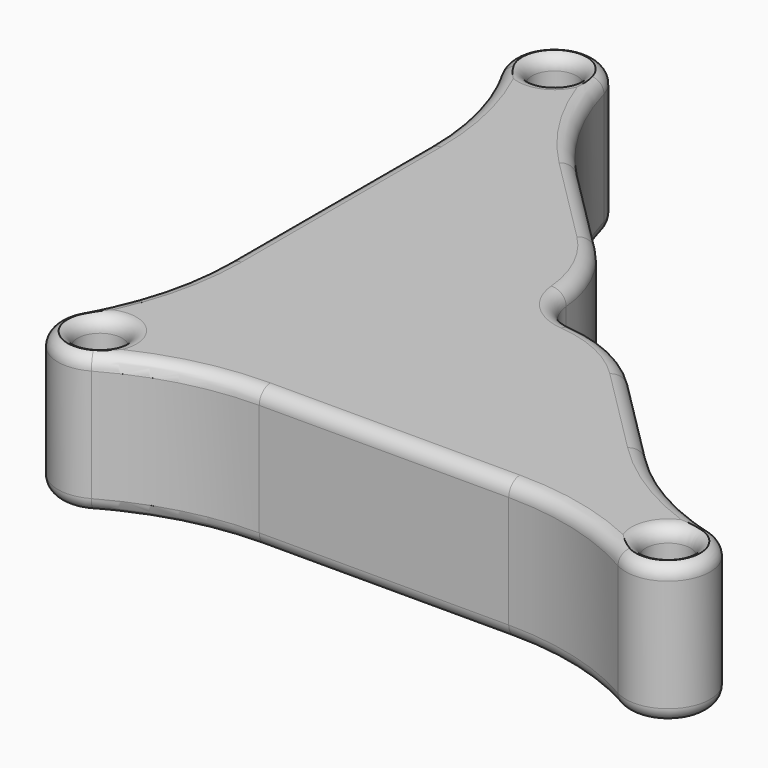
from build123d import *

# Parameters (mm, degrees)
F0_R          = 1.6
F1_DEPTH      = 10
F2_T3_ANGLE   = 29.591845794
F2_T6_ANGLE   = 194.1836915879
F2_T9_ANGLE   = 29.591845794
F2_T12_DEPTH  = 17.7843666168
F2_T15_ANGLE  = 29.591845794
F2_T18_ANGLE  = 149.1836915879
F2_T21_ANGLE  = 29.591845794
F2_T24_DEPTH  = 17.7843666168
F2_T27_ANGLE  = 29.591845794
F2_T30_ANGLE  = 194.1836915879
F2_T33_ANGLE  = 29.591845794
F2_T36_DEPTH  = 8.9733840835
F2_T39_ANGLE  = 39.7151372318
F2_T42_ANGLE  = 79.4302744637
F2_T45_ANGLE  = 39.7151372318
F2_T48_DEPTH  = 8.9733840835
F2_T60_ANGLE  = 29.591845794
F2_T63_ANGLE  = 194.1836915879
F2_T66_ANGLE  = 29.591845794
F2_T69_DEPTH  = 17.7843666168
F2_T72_ANGLE  = 29.591845794
F2_T75_ANGLE  = 149.1836915879
F2_T78_ANGLE  = 29.591845794
F2_T81_DEPTH  = 17.7843666168
F2_T84_ANGLE  = 29.591845794
F2_T87_ANGLE  = 194.1836915879
F2_T90_ANGLE  = 29.591845794
F2_T93_DEPTH  = 8.9733840835
F2_T96_ANGLE  = 39.7151372318
F2_T99_ANGLE  = 79.4302744637
F2_T102_ANGLE = 39.7151372318
F2_T105_DEPTH = 8.9733840835


# Not quite as in the source:
# - a fillet or chamfer that OpenCascade refuses, or shapes differently, is made with other operations: its cross-section is extruded or revolved along the edge and cut away or added


with BuildPart() as f1:
    # F0 (on Top) → F1 (new body)
    with BuildSketch(Plane.XY):
        with BuildLine():
            Line((11.3578166916, 0), (29.1421833084, 0))
            ThreePointArc((29.1421833084, 0), (34.249722493, -0.6631687322), (39.0185456489, -2.6086956522))
            ThreePointArc((39.0185456489, -2.6086956522), (43.2716385975, -1.1480502971), (41.297079968, 2.8921728034))
            ThreePointArc((41.297079968, 2.8921728034), (36.5493174981, 4.8885447172), (32.4688107979, 8.0311892021))
            Line((32.4688107979, 8.0311892021), (26.1236700622, 14.3763299378))
            ThreePointArc((26.1236700622, 14.3763299378), (23.3013016609, 16.3578061506), (19.9736774424, 17.2627527983))
            ThreePointArc((19.9736774424, 17.2627527983), (18.1286796564, 18.1286796564), (17.2627527983, 19.9736774424))
            ThreePointArc((17.2627527983, 19.9736774424), (16.3578061506, 23.3013016609), (14.3763299378, 26.1236700622))
            Line((14.3763299378, 26.1236700622), (8.0311892021, 32.4688107979))
            ThreePointArc((8.0311892021, 32.4688107979), (4.8885447172, 36.5493174981), (2.8921728034, 41.297079968))
            ThreePointArc((2.8921728034, 41.297079968), (-1.1480502971, 43.2716385975), (-2.6086956522, 39.0185456489))
            ThreePointArc((-2.6086956522, 39.0185456489), (-0.6631687322, 34.249722493), (0, 29.1421833084))
            Line((0, 29.1421833084), (0, 11.3578166916))
            ThreePointArc((0, 11.3578166916), (-0.6631687322, 6.250277507), (-2.6086956522, 1.4814543511))
            ThreePointArc((-2.6086956522, 1.4814543511), (-2.1213203436, -2.1213203436), (1.4814543511, -2.6086956522))
            ThreePointArc((1.4814543511, -2.6086956522), (6.250277507, -0.6631687322), (11.3578166916, 0))
        make_face()
        Circle(F0_R, mode=Mode.SUBTRACT)
        with Locations((40.5, 0)):
            Circle(F0_R, mode=Mode.SUBTRACT)
        with Locations((0, 40.5)):
            Circle(F0_R, mode=Mode.SUBTRACT)
    extrude(amount=F1_DEPTH)

    # F2: fillet of radius 1 on 38 edges, made by hand


with BuildPart() as f2_tool1:
    # F2_s2 → F2_t3 (revolve)
    with BuildSketch(Plane(origin=(-12.2188107979, 12.2188107979, 0), x_dir=(0, 0, 1), z_dir=(0.7071067812, -0.7071067812, 0))):
        with BuildLine():
            ThreePointArc((9, -28.6378246381), (9.7071067812, -28.3449314192), (10, -27.6378246381))
            Line((10, -27.6378246381), (10, -28.6378246381))
            Line((10, -28.6378246381), (9, -28.6378246381))
        make_face()
    revolve(axis=Axis((22.1733248258, 46.6109464216, 10), (0, 0, -1)), revolution_arc=F2_T3_ANGLE)


with BuildPart() as f2_tool4:
    # F2_s5 → F2_t6 (revolve)
    with BuildSketch(Plane(origin=(-10.3738185255, 37.6409858605, 0), x_dir=(0, 0, 1), z_dir=(0.2656933227, -0.9640576011, 0))):
        with BuildLine():
            ThreePointArc((9, -13.7605795685), (9.7071067812, -13.4676863497), (10, -12.7605795685))
            Line((10, -12.7605795685), (10, -13.7605795685))
            Line((10, -13.7605795685), (9, -13.7605795685))
        make_face()
    revolve(axis=Axis((0, 40.5, 10), (0, 0, 1)), revolution_arc=F2_T6_ANGLE)


with BuildPart() as f2_tool7:
    # F2_s8 → F2_t9 (revolve)
    with BuildSketch(Plane(origin=(-17.3909858605, 30.6238185255, 0), x_dir=(0, 0, 1), z_dir=(-0.493818117, 0.8695652174, 0))):
        with BuildLine():
            ThreePointArc((9, 16.9996337396), (9.7071067812, 17.2925269584), (10, 17.9996337396))
            Line((10, 17.9996337396), (10, 16.9996337396))
            Line((10, 16.9996337396), (9, 16.9996337396))
        make_face()
    revolve(axis=Axis((-20, 29.1421833084, 10), (0, 0, -1)), revolution_arc=F2_T9_ANGLE)


with BuildPart() as f2_tool10:
    # F2_s11 → F2_t12 (new body)
    with BuildSketch(Plane.XZ.offset(-29.1421833084)):
        with BuildLine():
            ThreePointArc((0, 9), (0.2928932188, 9.7071067812), (1, 10))
            Line((1, 10), (0, 10))
            Line((0, 10), (0, 9))
        make_face()
    extrude(amount=F2_T12_DEPTH)


with BuildPart() as f2_tool13:
    # F2_s14 → F2_t15 (revolve)
    with BuildSketch(Plane.XZ.offset(-11.3578166916)):
        with BuildLine():
            ThreePointArc((0, 9), (0.2928932188, 9.7071067812), (1, 10))
            Line((1, 10), (0, 10))
            Line((0, 10), (0, 9))
        make_face()
    revolve(axis=Axis((-20, 11.3578166916, 10), (0, 0, -1)), revolution_arc=F2_T15_ANGLE)


with BuildPart() as f2_tool16:
    # F2_s17 → F2_t18 (revolve)
    with BuildSketch(Plane(origin=(0, 0, 0), x_dir=(0, 0, 1), z_dir=(0.493818117, 0.8695652174, 0))):
        with BuildLine():
            ThreePointArc((9, -3), (9.7071067812, -2.7071067812), (10, -2))
            Line((10, -2), (10, -3))
            Line((10, -3), (9, -3))
        make_face()
    revolve(axis=Axis((0, 0, 10), (0, 0, 1)), revolution_arc=F2_T18_ANGLE)


with BuildPart() as f2_tool19:
    # F2_s20 → F2_t21 (revolve)
    with BuildSketch(Plane(origin=(0, 0, 0), x_dir=(0, 0, 1), z_dir=(-0.8695652174, -0.493818117, 0))):
        with BuildLine():
            ThreePointArc((9, -3), (9.7071067812, -2.7071067812), (10, -2))
            Line((10, -2), (10, -3))
            Line((10, -3), (9, -3))
        make_face()
    revolve(axis=Axis((11.3578166916, -20, 10), (0, 0, -1)), revolution_arc=F2_T21_ANGLE)


with BuildPart() as f2_tool22:
    # F2_s23 → F2_t24 (new body)
    with BuildSketch(Plane.YZ.offset(11.3578166916)):
        with BuildLine():
            ThreePointArc((0, 9), (0.2928932188, 9.7071067812), (1, 10))
            Line((1, 10), (0, 10))
            Line((0, 10), (0, 9))
        make_face()
    extrude(amount=F2_T24_DEPTH)


with BuildPart() as f2_tool25:
    # F2_s26 → F2_t27 (revolve)
    with BuildSketch(Plane.YZ.offset(29.1421833084)):
        with BuildLine():
            ThreePointArc((0, 9), (0.2928932188, 9.7071067812), (1, 10))
            Line((1, 10), (0, 10))
            Line((0, 10), (0, 9))
        make_face()
    revolve(axis=Axis((29.1421833084, -20, 10), (0, 0, -1)), revolution_arc=F2_T27_ANGLE)


with BuildPart() as f2_tool28:
    # F2_s29 → F2_t30 (revolve)
    with BuildSketch(Plane(origin=(30.6238185255, -17.3909858605, 0), x_dir=(0, 0, 1), z_dir=(-0.8695652174, 0.493818117, 0))):
        with BuildLine():
            ThreePointArc((9, 16.9996337396), (9.7071067812, 17.2925269584), (10, 17.9996337396))
            Line((10, 17.9996337396), (10, 16.9996337396))
            Line((10, 16.9996337396), (9, 16.9996337396))
        make_face()
    revolve(axis=Axis((40.5, 0, 10), (0, 0, 1)), revolution_arc=F2_T30_ANGLE)


with BuildPart() as f2_tool31:
    # F2_s32 → F2_t33 (revolve)
    with BuildSketch(Plane(origin=(37.6409858605, -10.3738185255, 0), x_dir=(0, 0, 1), z_dir=(0.9640576011, -0.2656933227, 0))):
        with BuildLine():
            ThreePointArc((9, -13.7605795685), (9.7071067812, -13.4676863497), (10, -12.7605795685))
            Line((10, -12.7605795685), (10, -13.7605795685))
            Line((10, -13.7605795685), (9, -13.7605795685))
        make_face()
    revolve(axis=Axis((46.6109464216, 22.1733248258, 10), (0, 0, -1)), revolution_arc=F2_T33_ANGLE)


with BuildPart() as f2_tool34:
    # F2_s35 → F2_t36 (new body)
    with BuildSketch(Plane(origin=(12.2188107979, -12.2188107979, 0), x_dir=(0, 0, 1), z_dir=(-0.7071067812, 0.7071067812, 0))):
        with BuildLine():
            ThreePointArc((9, 28.6378246381), (9.7071067812, 28.3449314192), (10, 27.6378246381))
            Line((10, 27.6378246381), (10, 28.6378246381))
            Line((10, 28.6378246381), (9, 28.6378246381))
        make_face()
    extrude(amount=F2_T36_DEPTH)


with BuildPart() as f2_tool37:
    # F2_s38 → F2_t39 (revolve)
    with BuildSketch(Plane(origin=(5.8736700622, -5.8736700622, 0), x_dir=(0, 0, 1), z_dir=(0.7071067812, -0.7071067812, 0))):
        with BuildLine():
            ThreePointArc((9, -28.6378246381), (9.7071067812, -28.3449314192), (10, -27.6378246381))
            Line((10, -27.6378246381), (10, -28.6378246381))
            Line((10, -28.6378246381), (9, -28.6378246381))
        make_face()
    revolve(axis=Axis((19.0526022504, 7.3052621259, 10), (0, 0, 1)), revolution_arc=F2_T39_ANGLE)


with BuildPart() as f2_tool40:
    # F2_s41 → F2_t42 (revolve)
    with BuildSketch(Plane(origin=(18.2209546286, -1.6854516701, 0), x_dir=(0, 0, 1), z_dir=(0.9957490672, -0.0921075192, 0))):
        with BuildLine():
            ThreePointArc((9, -19.0290958754), (9.7071067812, -18.7362026566), (10, -18.0290958754))
            Line((10, -18.0290958754), (10, -19.0290958754))
            Line((10, -19.0290958754), (9, -19.0290958754))
        make_face()
    revolve(axis=Axis((20.25, 20.25, 10), (0, 0, -1)), revolution_arc=F2_T42_ANGLE)


with BuildPart() as f2_tool43:
    # F2_s44 → F2_t45 (revolve)
    with BuildSketch(Plane(origin=(-1.6854516701, 18.2209546286, 0), x_dir=(0, 0, 1), z_dir=(0.0921075192, -0.9957490672, 0))):
        with BuildLine():
            ThreePointArc((9, -19.0290958754), (9.7071067812, -18.7362026566), (10, -18.0290958754))
            Line((10, -18.0290958754), (10, -19.0290958754))
            Line((10, -19.0290958754), (9, -19.0290958754))
        make_face()
    revolve(axis=Axis((7.3052621259, 19.0526022504, 10), (0, 0, 1)), revolution_arc=F2_T45_ANGLE)


with BuildPart() as f2_tool46:
    # F2_s47 → F2_t48 (new body)
    with BuildSketch(Plane(origin=(-5.8736700622, 5.8736700622, 0), x_dir=(0, 0, 1), z_dir=(-0.7071067812, 0.7071067812, 0))):
        with BuildLine():
            ThreePointArc((9, 28.6378246381), (9.7071067812, 28.3449314192), (10, 27.6378246381))
            Line((10, 27.6378246381), (10, 28.6378246381))
            Line((10, 28.6378246381), (9, 28.6378246381))
        make_face()
    extrude(amount=F2_T48_DEPTH)


with BuildPart() as f2_tool49:
    # F2_s50 → F2_t51 (revolve)
    with BuildSketch(Plane.XZ):
        with BuildLine():
            ThreePointArc((1.6, 9), (1.8928932188, 9.7071067812), (2.6, 10))
            Line((2.6, 10), (1.6, 10))
            Line((1.6, 10), (1.6, 9))
        make_face()
    revolve(axis=Axis((0, 0, 10), (0, 0, 1)))


with BuildPart() as f2_tool52:
    # F2_s53 → F2_t54 (revolve)
    with BuildSketch(Plane.XZ):
        with BuildLine():
            ThreePointArc((42.1, 9), (42.3928932188, 9.7071067812), (43.1, 10))
            Line((43.1, 10), (42.1, 10))
            Line((42.1, 10), (42.1, 9))
        make_face()
    revolve(axis=Axis((40.5, 0, 10), (0, 0, 1)))


with BuildPart() as f2_tool55:
    # F2_s56 → F2_t57 (revolve)
    with BuildSketch(Plane.XZ.offset(-40.5)):
        with BuildLine():
            ThreePointArc((1.6, 9), (1.8928932188, 9.7071067812), (2.6, 10))
            Line((2.6, 10), (1.6, 10))
            Line((1.6, 10), (1.6, 9))
        make_face()
    revolve(axis=Axis((0, 40.5, 10), (0, 0, 1)))


with BuildPart() as f2_tool58:
    # F2_s59 → F2_t60 (revolve)
    with BuildSketch(Plane(origin=(-12.2188107979, 12.2188107979, 0), x_dir=(0, 0, 1), z_dir=(0.7071067812, -0.7071067812, 0))):
        with BuildLine():
            ThreePointArc((1, -28.6378246381), (0.2928932188, -28.3449314192), (0, -27.6378246381))
            Line((0, -27.6378246381), (0, -28.6378246381))
            Line((0, -28.6378246381), (1, -28.6378246381))
        make_face()
    revolve(axis=Axis((22.1733248258, 46.6109464216, 0), (0, 0, -1)), revolution_arc=F2_T60_ANGLE)


with BuildPart() as f2_tool61:
    # F2_s62 → F2_t63 (revolve)
    with BuildSketch(Plane(origin=(-10.3738185255, 37.6409858605, 0), x_dir=(0, 0, 1), z_dir=(0.2656933227, -0.9640576011, 0))):
        with BuildLine():
            ThreePointArc((1, -13.7605795685), (0.2928932188, -13.4676863497), (0, -12.7605795685))
            Line((0, -12.7605795685), (0, -13.7605795685))
            Line((0, -13.7605795685), (1, -13.7605795685))
        make_face()
    revolve(axis=Axis((0, 40.5, 0), (0, 0, 1)), revolution_arc=F2_T63_ANGLE)


with BuildPart() as f2_tool64:
    # F2_s65 → F2_t66 (revolve)
    with BuildSketch(Plane(origin=(-17.3909858605, 30.6238185255, 0), x_dir=(0, 0, 1), z_dir=(-0.493818117, 0.8695652174, 0))):
        with BuildLine():
            ThreePointArc((1, 16.9996337396), (0.2928932188, 17.2925269584), (0, 17.9996337396))
            Line((0, 17.9996337396), (0, 16.9996337396))
            Line((0, 16.9996337396), (1, 16.9996337396))
        make_face()
    revolve(axis=Axis((-20, 29.1421833084, 0), (0, 0, -1)), revolution_arc=F2_T66_ANGLE)


with BuildPart() as f2_tool67:
    # F2_s68 → F2_t69 (new body)
    with BuildSketch(Plane.XZ.offset(-29.1421833084)):
        with BuildLine():
            ThreePointArc((0, 1), (0.2928932188, 0.2928932188), (1, 0))
            Line((1, 0), (0, 0))
            Line((0, 0), (0, 1))
        make_face()
    extrude(amount=F2_T69_DEPTH)


with BuildPart() as f2_tool70:
    # F2_s71 → F2_t72 (revolve)
    with BuildSketch(Plane.XZ.offset(-11.3578166916)):
        with BuildLine():
            ThreePointArc((0, 1), (0.2928932188, 0.2928932188), (1, 0))
            Line((1, 0), (0, 0))
            Line((0, 0), (0, 1))
        make_face()
    revolve(axis=Axis((-20, 11.3578166916, 0), (0, 0, -1)), revolution_arc=F2_T72_ANGLE)


with BuildPart() as f2_tool73:
    # F2_s74 → F2_t75 (revolve)
    with BuildSketch(Plane(origin=(0, 0, 0), x_dir=(0, 0, 1), z_dir=(0.493818117, 0.8695652174, 0))):
        with BuildLine():
            ThreePointArc((1, -3), (0.2928932188, -2.7071067812), (0, -2))
            Line((0, -2), (0, -3))
            Line((0, -3), (1, -3))
        make_face()
    revolve(axis=Axis((0, 0, 0), (0, 0, 1)), revolution_arc=F2_T75_ANGLE)


with BuildPart() as f2_tool76:
    # F2_s77 → F2_t78 (revolve)
    with BuildSketch(Plane(origin=(0, 0, 0), x_dir=(0, 0, 1), z_dir=(-0.8695652174, -0.493818117, 0))):
        with BuildLine():
            ThreePointArc((1, -3), (0.2928932188, -2.7071067812), (0, -2))
            Line((0, -2), (0, -3))
            Line((0, -3), (1, -3))
        make_face()
    revolve(axis=Axis((11.3578166916, -20, 0), (0, 0, -1)), revolution_arc=F2_T78_ANGLE)


with BuildPart() as f2_tool79:
    # F2_s80 → F2_t81 (new body)
    with BuildSketch(Plane.YZ.offset(11.3578166916)):
        with BuildLine():
            ThreePointArc((0, 1), (0.2928932188, 0.2928932188), (1, 0))
            Line((1, 0), (0, 0))
            Line((0, 0), (0, 1))
        make_face()
    extrude(amount=F2_T81_DEPTH)


with BuildPart() as f2_tool82:
    # F2_s83 → F2_t84 (revolve)
    with BuildSketch(Plane.YZ.offset(29.1421833084)):
        with BuildLine():
            ThreePointArc((0, 1), (0.2928932188, 0.2928932188), (1, 0))
            Line((1, 0), (0, 0))
            Line((0, 0), (0, 1))
        make_face()
    revolve(axis=Axis((29.1421833084, -20, 0), (0, 0, -1)), revolution_arc=F2_T84_ANGLE)


with BuildPart() as f2_tool85:
    # F2_s86 → F2_t87 (revolve)
    with BuildSketch(Plane(origin=(30.6238185255, -17.3909858605, 0), x_dir=(0, 0, 1), z_dir=(-0.8695652174, 0.493818117, 0))):
        with BuildLine():
            ThreePointArc((1, 16.9996337396), (0.2928932188, 17.2925269584), (0, 17.9996337396))
            Line((0, 17.9996337396), (0, 16.9996337396))
            Line((0, 16.9996337396), (1, 16.9996337396))
        make_face()
    revolve(axis=Axis((40.5, 0, 0), (0, 0, 1)), revolution_arc=F2_T87_ANGLE)


with BuildPart() as f2_tool88:
    # F2_s89 → F2_t90 (revolve)
    with BuildSketch(Plane(origin=(37.6409858605, -10.3738185255, 0), x_dir=(0, 0, 1), z_dir=(0.9640576011, -0.2656933227, 0))):
        with BuildLine():
            ThreePointArc((1, -13.7605795685), (0.2928932188, -13.4676863497), (0, -12.7605795685))
            Line((0, -12.7605795685), (0, -13.7605795685))
            Line((0, -13.7605795685), (1, -13.7605795685))
        make_face()
    revolve(axis=Axis((46.6109464216, 22.1733248258, 0), (0, 0, -1)), revolution_arc=F2_T90_ANGLE)


with BuildPart() as f2_tool91:
    # F2_s92 → F2_t93 (new body)
    with BuildSketch(Plane(origin=(12.2188107979, -12.2188107979, 0), x_dir=(0, 0, 1), z_dir=(-0.7071067812, 0.7071067812, 0))):
        with BuildLine():
            ThreePointArc((1, 28.6378246381), (0.2928932188, 28.3449314192), (0, 27.6378246381))
            Line((0, 27.6378246381), (0, 28.6378246381))
            Line((0, 28.6378246381), (1, 28.6378246381))
        make_face()
    extrude(amount=F2_T93_DEPTH)


with BuildPart() as f2_tool94:
    # F2_s95 → F2_t96 (revolve)
    with BuildSketch(Plane(origin=(5.8736700622, -5.8736700622, 0), x_dir=(0, 0, 1), z_dir=(0.7071067812, -0.7071067812, 0))):
        with BuildLine():
            ThreePointArc((1, -28.6378246381), (0.2928932188, -28.3449314192), (0, -27.6378246381))
            Line((0, -27.6378246381), (0, -28.6378246381))
            Line((0, -28.6378246381), (1, -28.6378246381))
        make_face()
    revolve(axis=Axis((19.0526022504, 7.3052621259, 0), (0, 0, 1)), revolution_arc=F2_T96_ANGLE)


with BuildPart() as f2_tool97:
    # F2_s98 → F2_t99 (revolve)
    with BuildSketch(Plane(origin=(18.2209546286, -1.6854516701, 0), x_dir=(0, 0, 1), z_dir=(0.9957490672, -0.0921075192, 0))):
        with BuildLine():
            ThreePointArc((1, -19.0290958754), (0.2928932188, -18.7362026566), (0, -18.0290958754))
            Line((0, -18.0290958754), (0, -19.0290958754))
            Line((0, -19.0290958754), (1, -19.0290958754))
        make_face()
    revolve(axis=Axis((20.25, 20.25, 0), (0, 0, -1)), revolution_arc=F2_T99_ANGLE)


with BuildPart() as f2_tool100:
    # F2_s101 → F2_t102 (revolve)
    with BuildSketch(Plane(origin=(-1.6854516701, 18.2209546286, 0), x_dir=(0, 0, 1), z_dir=(0.0921075192, -0.9957490672, 0))):
        with BuildLine():
            ThreePointArc((1, -19.0290958754), (0.2928932188, -18.7362026566), (0, -18.0290958754))
            Line((0, -18.0290958754), (0, -19.0290958754))
            Line((0, -19.0290958754), (1, -19.0290958754))
        make_face()
    revolve(axis=Axis((7.3052621259, 19.0526022504, 0), (0, 0, 1)), revolution_arc=F2_T102_ANGLE)


with BuildPart() as f2_tool103:
    # F2_s104 → F2_t105 (new body)
    with BuildSketch(Plane(origin=(-5.8736700622, 5.8736700622, 0), x_dir=(0, 0, 1), z_dir=(-0.7071067812, 0.7071067812, 0))):
        with BuildLine():
            ThreePointArc((1, 28.6378246381), (0.2928932188, 28.3449314192), (0, 27.6378246381))
            Line((0, 27.6378246381), (0, 28.6378246381))
            Line((0, 28.6378246381), (1, 28.6378246381))
        make_face()
    extrude(amount=F2_T105_DEPTH)


with BuildPart() as f2_tool106:
    # F2_s107 → F2_t108 (revolve)
    with BuildSketch(Plane.XZ):
        with BuildLine():
            ThreePointArc((1.6, 1), (1.8928932188, 0.2928932188), (2.6, 0))
            Line((2.6, 0), (1.6, 0))
            Line((1.6, 0), (1.6, 1))
        make_face()
    revolve(axis=Axis((0, 0, 0), (0, 0, 1)))


with BuildPart() as f2_tool109:
    # F2_s110 → F2_t111 (revolve)
    with BuildSketch(Plane.XZ):
        with BuildLine():
            ThreePointArc((42.1, 1), (42.3928932188, 0.2928932188), (43.1, 0))
            Line((43.1, 0), (42.1, 0))
            Line((42.1, 0), (42.1, 1))
        make_face()
    revolve(axis=Axis((40.5, 0, 0), (0, 0, 1)))


with BuildPart() as f2_tool112:
    # F2_s113 → F2_t114 (revolve)
    with BuildSketch(Plane.XZ.offset(-40.5)):
        with BuildLine():
            ThreePointArc((1.6, 1), (1.8928932188, 0.2928932188), (2.6, 0))
            Line((2.6, 0), (1.6, 0))
            Line((1.6, 0), (1.6, 1))
        make_face()
    revolve(axis=Axis((0, 40.5, 0), (0, 0, 1)))


with BuildPart() as f1_1:
    add(f1.part)

    # F2_t115: cut F2_tool1, F2_tool4, F2_tool7, F2_tool10, F2_tool13, F2_tool16, F2_tool19, F2_tool22, F2_tool25, F2_tool28, F2_tool31, F2_tool34, F2_tool37, F2_tool40, F2_tool43, F2_tool46, F2_tool49, F2_tool52, F2_tool55, F2_tool58, F2_tool61, F2_tool64, F2_tool67, F2_tool70, F2_tool73, F2_tool76, F2_tool79, F2_tool82, F2_tool85, F2_tool88, F2_tool91, F2_tool94, F2_tool97, F2_tool100, F2_tool103, F2_tool106, F2_tool109, F2_tool112
    add([f2_tool1.part, f2_tool4.part, f2_tool7.part, f2_tool10.part, f2_tool13.part, f2_tool16.part, f2_tool19.part, f2_tool22.part, f2_tool25.part, f2_tool28.part, f2_tool31.part, f2_tool34.part, f2_tool37.part, f2_tool40.part, f2_tool43.part, f2_tool46.part, f2_tool49.part, f2_tool52.part, f2_tool55.part, f2_tool58.part, f2_tool61.part, f2_tool64.part, f2_tool67.part, f2_tool70.part, f2_tool73.part, f2_tool76.part, f2_tool79.part, f2_tool82.part, f2_tool85.part, f2_tool88.part, f2_tool91.part, f2_tool94.part, f2_tool97.part, f2_tool100.part, f2_tool103.part, f2_tool106.part, f2_tool109.part, f2_tool112.part], mode=Mode.SUBTRACT)


solid = f1_1.part
